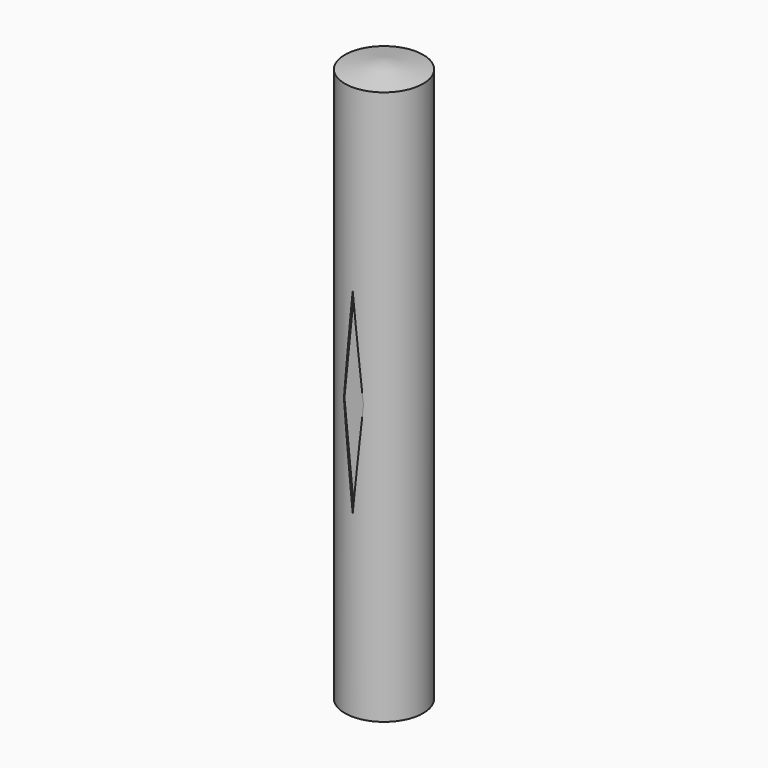
from build123d import *

# Parameters (mm, degrees)
F0_R       = 2
F1_DEPTH   = 29
F2_SIZE2   = 0.3526539614
F2_SIZE    = 2
F2_2_SIZE2 = 0.3526539614
F2_2_SIZE  = 2
F5_DEPTH   = 0.1


# Not quite as in the source:
# - a pattern or mirror of a feature is missing from the dataset's text; its kind, count and spacing are read off the source's solid


with BuildPart() as f1:
    # F0 (on Top) → F1 (new body)
    with BuildSketch(Plane.XY):
        Circle(F0_R)
    extrude(amount=F1_DEPTH)

    # F2
    f2_edges = [f1.edges().sort_by_distance(p)[0] for p in [
        (-2, 0, 29),
    ]]
    f2_side = f1.faces().sort_by_distance((0, 0, 29))[0]
    chamfer(f2_edges, length=F2_SIZE, length2=F2_SIZE2, reference=f2_side)

    # F2#2
    f2_2_edges = [f1.edges().sort_by_distance(p)[0] for p in [
        (-2, 0, 0),
    ]]
    f2_2_side = f1.faces().sort_by_distance((0, 0, 0))[0]
    chamfer(f2_2_edges, length=F2_2_SIZE, length2=F2_2_SIZE2, reference=f2_2_side)

    # F4 (on offset) → F5 (cut)
    with BuildSketch(Plane.XZ.offset(2)):
        Polygon((0.5, 14.5), (0, 19.5), (-0.5, 14.5), (0, 9.5), align=None)
    f5 = extrude(amount=-F5_DEPTH, mode=Mode.SUBTRACT)

    # F5_copies: F5 across plane
    add(f5.mirror(Plane.ZX), mode=Mode.SUBTRACT)


solid = f1.part
